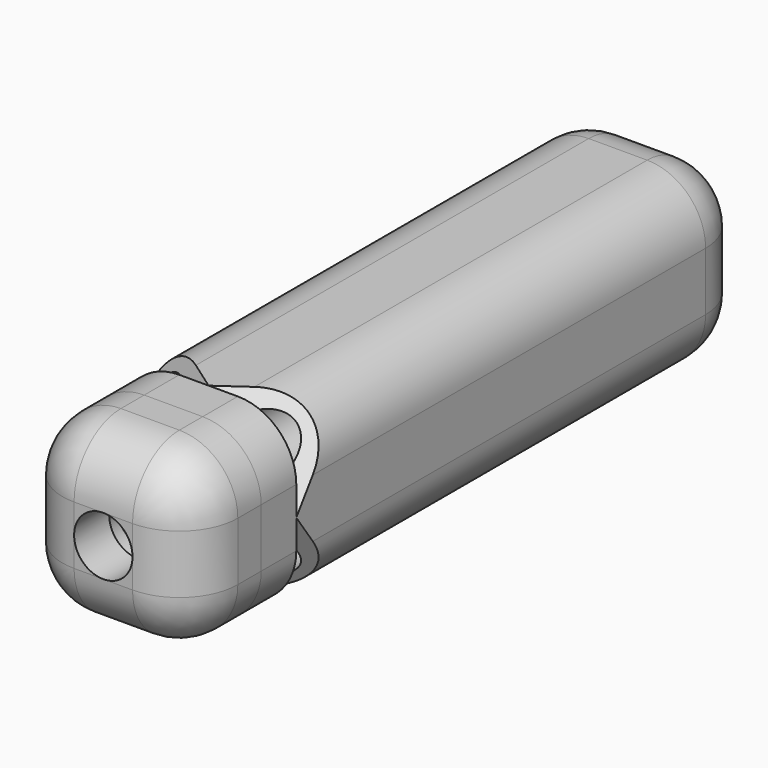
from build123d import *

# Parameters (mm, degrees)
F1_DEPTH  = 133.35
F3_D      = 12.7
F3_DEPTH  = 120.65
F3_TIP    = 3.8154649308
F4_D      = 12.7
F4_DEPTH  = 104.775
F4_TIP    = 3.8154649308
F5_D      = 12.7
F5_DEPTH  = 85.725
F5_TIP    = 3.8154649308
F6_D      = 12.7
F6_DEPTH  = 66.675
F6_TIP    = 3.8154649308
F11_DEPTH = 15.621
F14_DEPTH = 15.875
F17_DEPTH = 9.525
F20_DEPTH = 19.05
F21_R     = 17.4625
F22_DEPTH = 9.525
F24_D     = 12.7
F24_DEPTH = 9.525
F24_TIP   = 3.8154649308
F26_R     = 12.69999
F26_2_R   = 12.69999


# Not quite as in the source:
# - a fillet or chamfer is up to 0.001 mm smaller than in the source, because OpenCascade refuses the exact size
# - a feature of the source that left no trace in its solid (it failed there, or was rolled back) is left out


with BuildPart() as f1:
    # F0 (on Front) → F1 (new body)
    with BuildSketch(Plane.XZ):
        with BuildLine():
            ThreePointArc((19.05, 6.35), (15.3302561211, 15.3302561211), (6.35, 19.05))
            Line((6.35, 19.05), (-6.35, 19.05))
            ThreePointArc((-6.35, 19.05), (-15.3302561211, 15.3302561211), (-19.05, 6.35))
            Line((-19.05, 6.35), (-19.05, -6.35))
            ThreePointArc((-19.05, -6.35), (-15.3302561211, -15.3302561211), (-6.35, -19.05))
            Line((-6.35, -19.05), (6.35, -19.05))
            ThreePointArc((6.35, -19.05), (15.3302561211, -15.3302561211), (19.05, -6.35))
            Line((19.05, -6.35), (19.05, 6.35))
        make_face()
    extrude(amount=F1_DEPTH)

    # F3
    with Locations(Plane.XZ.offset(133.35)):
        with Locations((-9.525, -9.525)):
            Hole(F3_D / 2, depth=F3_DEPTH)
            with Locations((0, 0, -(F3_DEPTH + F3_TIP / 2))):  # 118° drill point
                Cone(0, F3_D / 2, F3_TIP, mode=Mode.SUBTRACT)

    # F4
    with Locations(Plane.XZ.offset(133.35)):
        with Locations((9.525, 9.525)):
            Hole(F4_D / 2, depth=F4_DEPTH)
            with Locations((0, 0, -(F4_DEPTH + F4_TIP / 2))):  # 118° drill point
                Cone(0, F4_D / 2, F4_TIP, mode=Mode.SUBTRACT)

    # F5
    with Locations(Plane.XZ.offset(133.35)):
        with Locations((-9.525, 9.525)):
            Hole(F5_D / 2, depth=F5_DEPTH)
            with Locations((0, 0, -(F5_DEPTH + F5_TIP / 2))):  # 118° drill point
                Cone(0, F5_D / 2, F5_TIP, mode=Mode.SUBTRACT)

    # F6
    with Locations(Plane.XZ.offset(133.35)):
        with Locations((9.525, -9.525)):
            Hole(F6_D / 2, depth=F6_DEPTH)
            with Locations((0, 0, -(F6_DEPTH + F6_TIP / 2))):  # 118° drill point
                Cone(0, F6_D / 2, F6_TIP, mode=Mode.SUBTRACT)

    # F10 (on line) → F11 (cut, symmetric)
    with BuildSketch(Plane(origin=(0, 0, 0), x_dir=(0, 1, 0), z_dir=(0.7071067812, 0, 0.7071067812))):
        Polygon((-123.825, 64.2703841816), (-123.825, 13.4703841816), (-73.025, 64.2703841816), align=None)
        Polygon((-123.825, -64.2703841816), (-73.025, -64.2703841816), (-123.825, -13.4703841816), align=None)
    extrude(amount=F11_DEPTH, both=True, mode=Mode.SUBTRACT)

    # F13 (on line) → F14 (cut, symmetric)
    with BuildSketch(Plane(origin=(0, 0, 0), x_dir=(0.7071067812, 0, 0.7071067812), z_dir=(0.7071067812, 0, -0.7071067812))):
        Polygon((38.8747, 123.825), (13.4747, 123.825), (38.8747, 98.425), align=None)
        Polygon((-38.8747, 123.825), (-38.8747, 98.425), (-13.4747, 123.825), align=None)
    extrude(amount=F14_DEPTH, both=True, mode=Mode.SUBTRACT)

    # F26 (radius 12.7 in the source; OpenCascade refuses exactly that, so slightly less here)
    f26_edges = [f1.edges().sort_by_distance(p)[0] for p in [
        (0, 0, 19.05),
        (19.05, 0, 0),
        (15.330256, 0, 15.330256),
        (-15.330256, 0, 15.330256),
        (-19.05, 0, 0),
        (-15.330256, 0, -15.330256),
        (0, 0, -19.05),
        (15.330256, 0, -15.330256),
    ]]
    fillet(f26_edges, radius=F26_R)


with BuildPart() as f17:
    # F16 (on offset) → F17 (new body)
    with BuildSketch(Plane.XZ.offset(133.35)):
        with BuildLine():
            Line((-5.0348719395, 14.0151280605), (-14.0151280605, 5.0348719395))
            ThreePointArc((-14.0151280605, 5.0348719395), (-5.0348719395, 5.0348719395), (-5.0348719395, 14.0151280605))
        make_face()
    extrude(amount=-F17_DEPTH)


with BuildPart() as f17b:
    # F16 (on offset) → F17, piece 2 (new body)
    with BuildSketch(Plane.XZ.offset(133.35)):
        with BuildLine():
            Line((14.0151280605, 5.0348719395), (5.0348719395, 14.0151280605))
            ThreePointArc((5.0348719395, 14.0151280605), (5.0348719395, 5.0348719395), (14.0151280605, 5.0348719395))
        make_face()
    extrude(amount=-F17_DEPTH)


with BuildPart() as f17c:
    # F16 (on offset) → F17, piece 3 (new body)
    with BuildSketch(Plane.XZ.offset(133.35)):
        with BuildLine():
            Line((5.0348719395, -14.0151280605), (14.0151280605, -5.0348719395))
            ThreePointArc((14.0151280605, -5.0348719395), (5.0348719395, -5.0348719395), (5.0348719395, -14.0151280605))
        make_face()
    extrude(amount=-F17_DEPTH)


with BuildPart() as f17d:
    # F16 (on offset) → F17, piece 4 (new body)
    with BuildSketch(Plane.XZ.offset(133.35)):
        with BuildLine():
            Line((-14.0151280605, -5.0348719395), (-5.0348719395, -14.0151280605))
            ThreePointArc((-5.0348719395, -14.0151280605), (-5.0348719395, -5.0348719395), (-14.0151280605, -5.0348719395))
        make_face()
    extrude(amount=-F17_DEPTH)


with BuildPart() as f20:
    # F19 (on offset) → F20 (new body)
    with BuildSketch(Plane.XZ.offset(152.4)):
        with BuildLine():
            Line((-6.35, -19.05), (6.35, -19.05))
            ThreePointArc((6.35, -19.05), (15.3302561211, -15.3302561211), (19.05, -6.35))
            Line((19.05, -6.35), (19.05, 6.35))
            ThreePointArc((19.05, 6.35), (15.3302561211, 15.3302561211), (6.35, 19.05))
            Line((6.35, 19.05), (-6.35, 19.05))
            ThreePointArc((-6.35, 19.05), (-15.3302561211, 15.3302561211), (-19.05, 6.35))
            Line((-19.05, 6.35), (-19.05, -6.35))
            ThreePointArc((-19.05, -6.35), (-15.3302561211, -15.3302561211), (-6.35, -19.05))
        make_face()
    extrude(amount=-F20_DEPTH)

    # F21 (on face) → F22 (cut)
    with BuildSketch(Plane(origin=(0, -133.35, 0), x_dir=(-1, 0, 0), z_dir=(0, 1, 0))):
        Circle(F21_R)
    extrude(amount=-F22_DEPTH, mode=Mode.SUBTRACT)

    # F24
    with Locations(Plane.XZ.offset(152.4)):
        with Locations((0, 0)):
            Hole(F24_D / 2, depth=F24_DEPTH)
            with Locations((0, 0, -(F24_DEPTH + F24_TIP / 2))):  # 118° drill point
                Cone(0, F24_D / 2, F24_TIP, mode=Mode.SUBTRACT)

    # F26#2 (radius 12.7 in the source; OpenCascade refuses exactly that, so slightly less here)
    f26_2_edges = [f20.edges().sort_by_distance(p)[0] for p in [
        (0, -152.4, 19.05),
        (-19.05, -152.4, 0),
        (-15.330256, -152.4, 15.330256),
        (-15.330256, -152.4, -15.330256),
        (0, -152.4, -19.05),
        (15.330256, -152.4, 15.330256),
        (15.330256, -152.4, -15.330256),
        (19.05, -152.4, 0),
    ]]
    fillet(f26_2_edges, radius=F26_2_R)


solid = Compound([f1.part, f17.part, f17b.part, f17c.part, f17d.part, f20.part])
